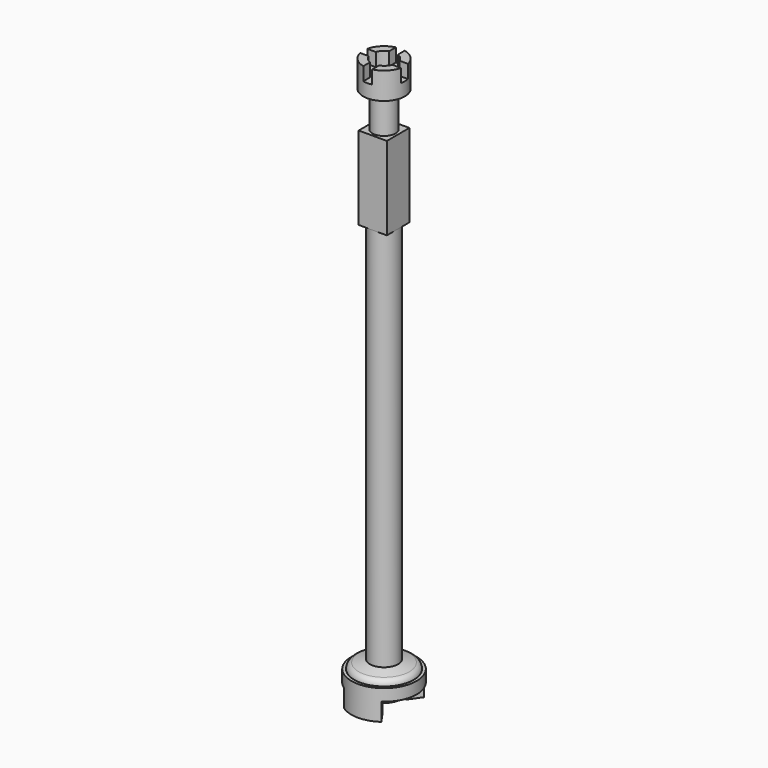
from build123d import *

# Parameters (mm, degrees)
F3_DEPTH        = 38.1
F4_DEPTH        = 76.2
F5_DEPTH        = 60.325
F8_DEPTH        = 57.15
F8_COPIES_COUNT = 4


# Not quite as in the source:
# - a pattern or mirror of a feature is missing from the dataset's text; its kind, count and spacing are read off the source's solid


with BuildPart() as f1:
    # F0 (on Front) → F1 (revolve)
    with BuildSketch(Plane.XZ):
        with BuildLine():
            Line((0, 1803.4), (0, 0))
            Line((0, 0), (139.7, 0))
            Line((139.7, 0), (139.7, 127))
            Line((139.7, 127), (127, 127))
            ThreePointArc((127, 127), (121.7511748434, 142.4625402968), (108.1740037456, 151.5345159877))
            Line((108.1740037456, 151.5345159877), (60.325, 164.3556179))
            Line((60.325, 164.3556179), (60.325, 1803.4))
            Line((60.325, 1803.4), (0, 1803.4))
        make_face()
    revolve(axis=Axis((0, 0, 901.7), (0, 0, -1)))

    # F2 (on face) → F3 (cut)
    with BuildSketch(Plane(origin=(0, 0, 0), x_dir=(1, 0, 0), z_dir=(0, 0, -1))):
        with BuildLine():
            ThreePointArc((43.7065244499, -62.4193857748), (67.5902254882, -35.1852443285), (76.2, 0))
            ThreePointArc((76.2, 0), (67.5902254882, 35.1852443285), (43.7065244499, 62.4193857748))
            ThreePointArc((43.7065244499, 62.4193857748), (0, 76.2), (-43.7065244499, 62.4193857748))
            ThreePointArc((-43.7065244499, 62.4193857748), (-76.2, 0), (-43.7065244499, -62.4193857748))
            ThreePointArc((-43.7065244499, -62.4193857748), (0, -76.2), (43.7065244499, -62.4193857748))
        make_face()
    extrude(amount=-F3_DEPTH, mode=Mode.SUBTRACT)

    # F2 (on face) → F4 (cut)
    with BuildSketch(Plane(origin=(0, 0, 0), x_dir=(1, 0, 0), z_dir=(0, 0, -1))):
        with BuildLine():
            ThreePointArc((-43.7065244499, -62.4193857748), (-76.2, 0), (-43.7065244499, 62.4193857748))
            Line((-43.7065244499, 62.4193857748), (-80.1286281582, 114.4355405872))
            ThreePointArc((-80.1286281582, 114.4355405872), (-139.7, 0), (-80.1286281582, -114.4355405872))
            Line((-80.1286281582, -114.4355405872), (-43.7065244499, -62.4193857748))
        make_face()
        with BuildLine():
            ThreePointArc((43.7065244499, 62.4193857748), (67.5902254882, 35.1852443285), (76.2, 0))
            ThreePointArc((76.2, 0), (67.5902254882, -35.1852443285), (43.7065244499, -62.4193857748))
            Line((43.7065244499, -62.4193857748), (80.1286281582, -114.4355405872))
            ThreePointArc((80.1286281582, -114.4355405872), (123.915413395, -64.5062812689), (139.7, 0))
            ThreePointArc((139.7, 0), (123.915413395, 64.5062812689), (80.1286281582, 114.4355405872))
            Line((80.1286281582, 114.4355405872), (43.7065244499, 62.4193857748))
        make_face()
    extrude(amount=-F4_DEPTH, mode=Mode.SUBTRACT)

    # F0 (on Front) → F5 (join, symmetric)
    with BuildSketch(Plane.XZ):
        Polygon((-60.325, 1803.4), (0, 1803.4), (60.325, 1803.4), (60.325, 2159), (49.2125, 2159), (0, 2159), (-60.325, 2159), align=None)
    extrude(amount=F5_DEPTH, both=True)

    # F0 (on Front) → F6 (revolve)
    with BuildSketch(Plane.XZ):
        Polygon((0, 2159), (49.2125, 2159), (49.2125, 2311.4), (88.9, 2311.4), (88.9, 2425.7), (53.975, 2425.7), (53.975, 2368.55), (0, 2368.55), align=None)
    revolve(axis=Axis((0, 0, 2263.775), (0, 0, -1)))

    # F7 (on face) → F8 (cut, through all)
    with BuildSketch(Plane.XY.offset(2425.7)):
        with BuildLine():
            ThreePointArc((53.975, 0), (53.0995163948, -9.6820443933), (50.5014665629, -19.05))
            Line((50.5014665629, -19.05), (86.834944003, -19.05))
            ThreePointArc((86.834944003, -19.05), (88.3822281962, -9.5808005442), (88.9, 0))
            ThreePointArc((88.9, 0), (88.3822281962, 9.5808005442), (86.834944003, 19.05))
            Line((86.834944003, 19.05), (50.5014665629, 19.05))
            ThreePointArc((50.5014665629, 19.05), (53.0995163948, 9.6820443933), (53.975, 0))
        make_face()
    f8 = extrude(amount=-F8_DEPTH, mode=Mode.SUBTRACT)

    # F8_copies: F8 ×4 about axis
    f8_copies_axis = Axis((0, 0, 0), (0, 0, 1))
    for i in range(1, F8_COPIES_COUNT):
        add(f8.rotate(f8_copies_axis, i * 360 / F8_COPIES_COUNT), mode=Mode.SUBTRACT)


solid = f1.part
